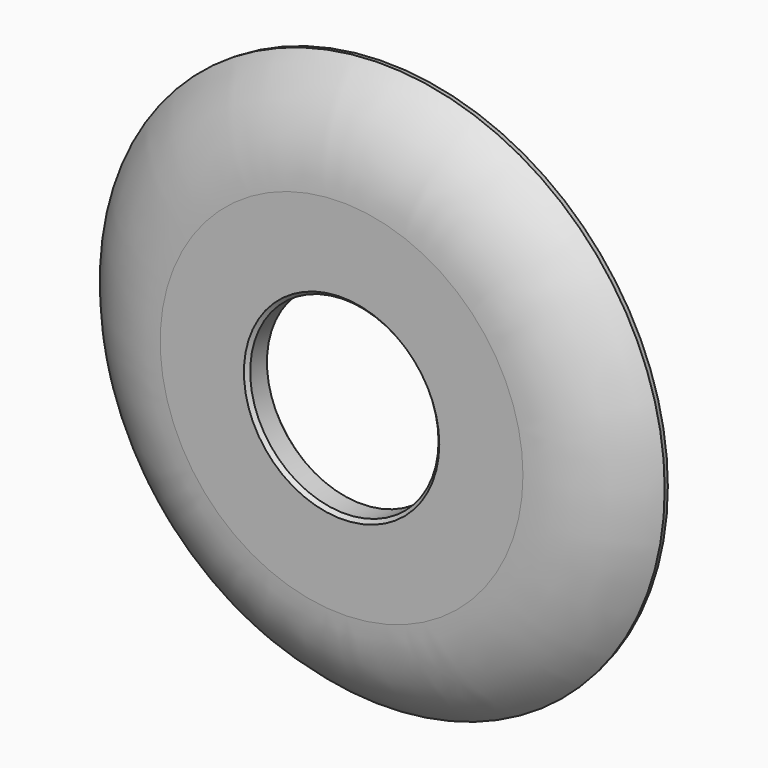
from build123d import *


# Not quite as in the source:
# - a fillet or chamfer that OpenCascade refuses, or shapes differently, is made with other operations: its cross-section is extruded or revolved along the edge and cut away or added


with BuildPart() as f1:
    # F0 (on Top) → F1 (revolve)
    with BuildSketch(Plane.XY):
        with BuildLine():
            Line((26, 4), (13.5, 4))
            Line((13.5, 4), (13.5, 0))
            Line((13.5, 0), (26, 0))
            ThreePointArc((26, 0), (34.3358249123, 2.0438355847), (40.7808320951, 7.7117384844))
            Line((40.7808320951, 7.7117384844), (37.5, 10))
            ThreePointArc((37.5, 10), (32.4855608855, 5.5901749694), (26, 4))
        make_face()
    revolve(axis=Axis((0, 5.3547318093, 0), (0, 1, 0)))

    # F2: chamfer of 0.5 on 5 edges, made by hand

    # F2_s1 → F2_t2 (revolve, cut)
    with BuildSketch(Plane.XY):
        Polygon((14, 4), (13.5, 3.5), (13.5, 4), align=None)
    revolve(axis=Axis((0, 4, 0), (0, 1, 0)), mode=Mode.SUBTRACT)

    # F2_s3 → F2_t4 (revolve, cut)
    with BuildSketch(Plane.XY):
        Polygon((13.5, 0.5), (14, 0), (13.5, 0), align=None)
    revolve(axis=Axis((0, 0, 0), (0, 1, 0)), mode=Mode.SUBTRACT)

    # F2_s5 → F2_t6 (revolve, cut)
    with BuildSketch(Plane.XY):
        with BuildLine():
            Line((37.9030413035, 9.7188932937), (37.2169968397, 9.608773582))
            ThreePointArc((37.2169968397, 9.608773582), (37.3560341631, 9.7974365018), (37.5, 10))
            Line((37.5, 10), (37.9030413035, 9.7188932937))
        make_face()
    revolve(axis=Axis((0, 10, 0), (0, 1, 0)), mode=Mode.SUBTRACT)

    # F2_s7 → F2_t8 (revolve, cut)
    with BuildSketch(Plane.XY):
        with BuildLine():
            Line((40.4806168806, 7.2941297957), (40.3648752289, 8.0018533277))
            Line((40.3648752289, 8.0018533277), (40.7808320951, 7.7117384844))
            ThreePointArc((40.7808320951, 7.7117384844), (40.6280870104, 7.4961241001), (40.4806168806, 7.2941297957))
        make_face()
    revolve(axis=Axis((0, 7.7117384844, 0), (0, 1, 0)), mode=Mode.SUBTRACT)


solid = f1.part
